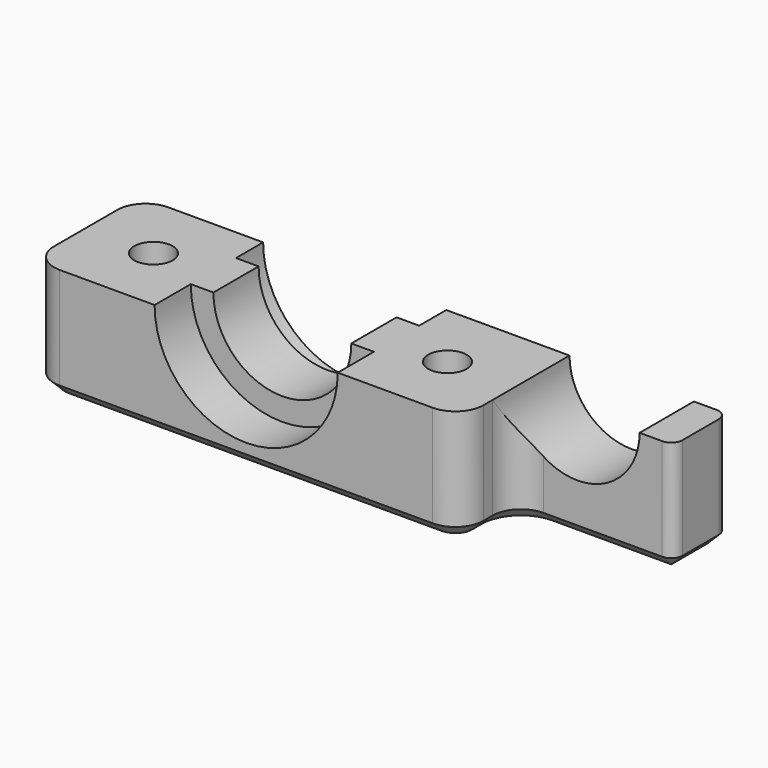
from build123d import *

# Parameters (mm, degrees)
F1_DEPTH      = 6
F2_DEPTH      = 2
F2_DEPTH_BACK = 3
F3_DEPTH      = 6
F4_R          = 2.9
F4_R_2        = 1.7
F5_DEPTH      = 3.5
F6_R          = 2.5
F7_T4_DEPTH   = 10
F7_S5_R       = 5.5
F7_T6_DEPTH   = 7
F7_T7_DEPTH   = 22.5
F8_R          = 1
F9_T1_DEPTH   = 48.4999999995
F9_T3_DEPTH   = 10.5
F9_T5_DEPTH   = 4
F9_T7_DEPTH   = 1
F9_T9_DEPTH   = 32.9999999994
F9_T11_DEPTH  = 7
F9_T18_ANGLE  = 90
F9_T20_ANGLE  = 89.9999999974
F9_T22_ANGLE  = 90
F9_T24_ANGLE  = 90.0000000053
F9_T26_ANGLE  = 90
F9_T28_ANGLE  = 90
F10_R         = 1.7
F11_DEPTH     = 6.4


# Not quite as in the source:
# - a fillet or chamfer that OpenCascade refuses, or shapes differently, is made with other operations: its cross-section is extruded or revolved along the edge and cut away or added


with BuildPart() as f1:
    # F0 (on Front) → F1 (new body, symmetric)
    with BuildSketch(Plane.XZ):
        with BuildLine():
            Line((18.9999999997, 0), (18.9999999997, 10))
            Line((18.9999999997, 10), (8.099, 10))
            ThreePointArc((8.099, 10), (0, 1.901), (-8.099, 10))
            Line((-8.099, 10), (-18.9999999997, 10))
            Line((-18.9999999997, 10), (-18.9999999997, 0))
            Line((-18.9999999997, 0), (18.9999999997, 0))
        make_face()
    extrude(amount=F1_DEPTH, both=True)

    # F0 (on Front) → F2 (join, two sides)
    with BuildSketch(Plane.XZ) as f2_sk:
        with BuildLine():
            ThreePointArc((-8.099, 10), (0, 1.901), (8.099, 10))
            Line((8.099, 10), (6.099, 10))
            ThreePointArc((6.099, 10), (0, 3.901), (-6.099, 10))
            Line((-6.099, 10), (-8.099, 10))
        make_face()
    extrude(amount=F2_DEPTH)
    extrude(f2_sk.sketch, amount=-F2_DEPTH_BACK)

    # F0 (on Front) → F3 (join)
    with BuildSketch(Plane.XZ):
        with BuildLine():
            ThreePointArc((29.9999999997, 10), (24.4999999997, 4.5), (18.9999999997, 10))
            Line((18.9999999997, 10), (18.9999999997, 0))
            Line((18.9999999997, 0), (32.9999999997, 0))
            Line((32.9999999997, 0), (32.9999999997, 10))
            Line((32.9999999997, 10), (29.9999999997, 10))
        make_face()
    extrude(amount=-F3_DEPTH)

    # F4 (on face) → F5 (cut)
    with BuildSketch(Plane(origin=(0, 0, 0), x_dir=(1, 0, 0), z_dir=(0, 0, -1))):
        with Locations((13, 0)):
            Circle(F4_R)
        with Locations((13, 0)):
            Circle(F4_R_2, mode=Mode.SUBTRACT)
        with Locations((-13, 0)):
            Circle(F4_R)
        with Locations((-13, 0)):
            Circle(F4_R_2, mode=Mode.SUBTRACT)
        with Locations((13, 0)):
            Circle(F4_R_2)
        with Locations((-13, 0)):
            Circle(F4_R_2)
    extrude(amount=-F5_DEPTH, mode=Mode.SUBTRACT)

    # F6
    f6_edges = [f1.edges().sort_by_distance(p)[0] for p in [
        (-19, 6, 5),
        (-19, -6, 5),
    ]]
    fillet(f6_edges, radius=F6_R)

    # F7: fillet of radius 2.5 on 2 edges, made by hand


with BuildPart() as f7_tool2:
    # F7_s3 → F7_t4 (new body)
    with BuildSketch(Plane.XY.offset(10)):
        with BuildLine():
            ThreePointArc((21.4999999997, 0), (19.7322330468, -0.732233047), (18.9999999997, -2.5))
            Line((18.9999999997, -2.5), (18.9999999997, 0))
            Line((18.9999999997, 0), (21.4999999997, 0))
        make_face()
    extrude(amount=-F7_T4_DEPTH)

    # F7_s5 → F7_t6 (cut, symmetric)
    with BuildSketch(Plane.XZ.offset(1.2)):
        with Locations((24.4999999997, 10)):
            Circle(F7_S5_R)
    extrude(amount=F7_T6_DEPTH, both=True, mode=Mode.SUBTRACT)


with BuildPart() as f1_1:
    add(f1.part)

    # F7_t1: union F7_tool2
    add(f7_tool2.part)

    # F7_s8 → F7_t7 (cut)
    with BuildSketch(Plane.XY.offset(-6.25)):
        with BuildLine():
            ThreePointArc((16.4999999997, -6), (18.2677669527, -5.267766953), (18.9999999997, -3.5))
            Line((18.9999999997, -3.5), (18.9999999997, -6))
            Line((18.9999999997, -6), (16.4999999997, -6))
        make_face()
    extrude(amount=F7_T7_DEPTH, mode=Mode.SUBTRACT)

    # F8
    f8_edges = [f1_1.edges().sort_by_distance(p)[0] for p in [
        (33, 6, 5),
        (33, 0, 5),
    ]]
    fillet(f8_edges, radius=F8_R)

    # F9: chamfer of 1 on 14 edges, made by hand

    # F9_s2 → F9_t1 (cut)
    with BuildSketch(Plane.YZ.offset(-16.4999999997)):
        Polygon((5, 0), (6, 1), (6, 0), align=None)
    extrude(amount=F9_T1_DEPTH, mode=Mode.SUBTRACT)

    # F9_s4 → F9_t3 (cut)
    with BuildSketch(Plane.YZ.offset(21.4999999997)):
        Polygon((1, 0), (0, 1), (0, 0), align=None)
    extrude(amount=F9_T3_DEPTH, mode=Mode.SUBTRACT)

    # F9_s6 → F9_t5 (cut)
    with BuildSketch(Plane.XZ.offset(-5)):
        Polygon((31.9999999997, 0), (32.9999999997, 1), (32.9999999997, 0), align=None)
    extrude(amount=F9_T5_DEPTH, mode=Mode.SUBTRACT)

    # F9_s8 → F9_t7 (cut)
    with BuildSketch(Plane.XZ.offset(2.5)):
        Polygon((17.9999999997, 0), (18.9999999997, 1), (18.9999999997, 0), align=None)
    extrude(amount=F9_T7_DEPTH, mode=Mode.SUBTRACT)

    # F9_s10 → F9_t9 (cut)
    with BuildSketch(Plane.YZ.offset(-16.4999999997)):
        Polygon((-5, 0), (-6, 1), (-6, 0), align=None)
    extrude(amount=F9_T9_DEPTH, mode=Mode.SUBTRACT)

    # F9_s12 → F9_t11 (cut)
    with BuildSketch(Plane.XZ.offset(-3.5)):
        Polygon((-17.9999999997, 0), (-18.9999999997, 1), (-18.9999999997, 0), align=None)
    extrude(amount=F9_T11_DEPTH, mode=Mode.SUBTRACT)

    # F9_s13 → F9_t14 (revolve, cut)
    with BuildSketch(Plane.XZ):
        Polygon((-9.1, 0), (-10.1, 1), (-10.1, 0), align=None)
    revolve(axis=Axis((-13, 0, 0), (0, 0, -1)), mode=Mode.SUBTRACT)

    # F9_s15 → F9_t16 (revolve, cut)
    with BuildSketch(Plane.XZ):
        Polygon((16.9, 0), (15.9, 1), (15.9, 0), align=None)
    revolve(axis=Axis((13, 0, 0), (0, 0, -1)), mode=Mode.SUBTRACT)

    # F9_s17 → F9_t18 (revolve, cut)
    with BuildSketch(Plane.YZ.offset(31.9999999997)):
        Polygon((1, 0), (0, 1), (0, 0), align=None)
    revolve(axis=Axis((31.9999999997, 1, 0), (0, 0, 1)), revolution_arc=F9_T18_ANGLE, mode=Mode.SUBTRACT)

    # F9_s19 → F9_t20 (revolve, cut)
    with BuildSketch(Plane.YZ.offset(21.4999999998)):
        Polygon((1, 0), (0, 1), (0, 0), align=None)
    revolve(axis=Axis((21.4999999998, -2.5000000001, 0), (0, 0, 1)), revolution_arc=F9_T20_ANGLE, mode=Mode.SUBTRACT)

    # F9_s21 → F9_t22 (revolve, cut)
    with BuildSketch(Plane.XZ.offset(-5)):
        Polygon((31.9999999997, 0), (32.9999999997, 1), (32.9999999997, 0), align=None)
    revolve(axis=Axis((31.9999999997, 5, 0), (0, 0, 1)), revolution_arc=F9_T22_ANGLE, mode=Mode.SUBTRACT)

    # F9_s23 → F9_t24 (revolve, cut)
    with BuildSketch(Plane.XZ.offset(3.5000000001)):
        Polygon((17.9999999997, 0), (18.9999999997, 1), (18.9999999997, 0), align=None)
    revolve(axis=Axis((16.4999999998, -3.5000000001, 0), (0, 0, -1)), revolution_arc=F9_T24_ANGLE, mode=Mode.SUBTRACT)

    # F9_s25 → F9_t26 (revolve, cut)
    with BuildSketch(Plane.YZ.offset(-16.4999999997)):
        Polygon((5, 0), (6, 1), (6, 0), align=None)
    revolve(axis=Axis((-16.4999999997, 3.5, 0), (0, 0, 1)), revolution_arc=F9_T26_ANGLE, mode=Mode.SUBTRACT)

    # F9_s27 → F9_t28 (revolve, cut)
    with BuildSketch(Plane.XZ.offset(3.5)):
        Polygon((-17.9999999997, 0), (-18.9999999997, 1), (-18.9999999997, 0), align=None)
    revolve(axis=Axis((-16.4999999997, -3.5, 0), (0, 0, 1)), revolution_arc=F9_T28_ANGLE, mode=Mode.SUBTRACT)

    # F10 (on face) → F11 (cut)
    with BuildSketch(Plane.XY.offset(10)):
        with Locations((-13, 0)):
            Circle(F10_R)
        with Locations((13, 0)):
            Circle(F10_R)
    extrude(amount=-F11_DEPTH, mode=Mode.SUBTRACT)


solid = f1_1.part
